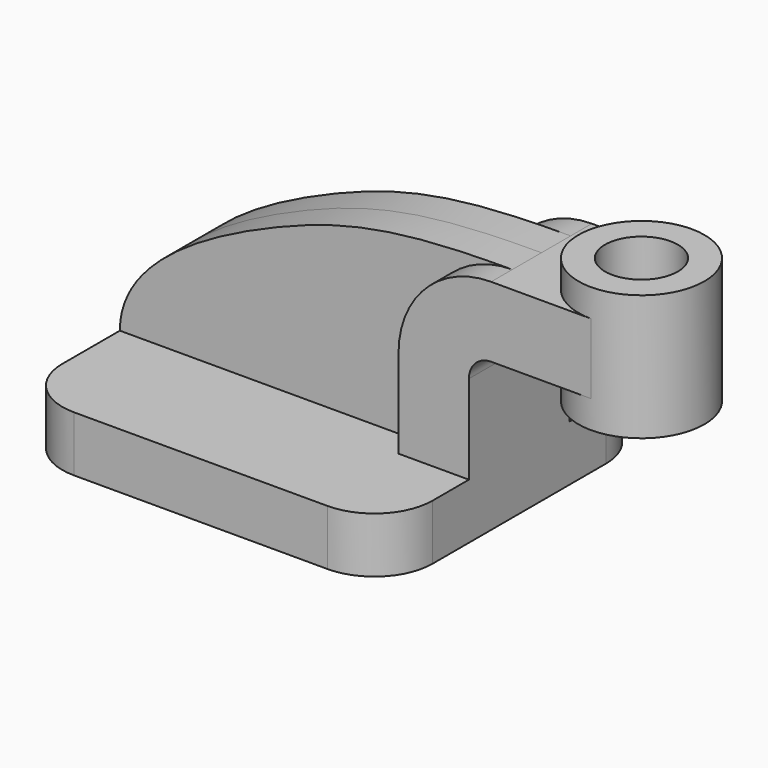
from build123d import *

# Parameters (mm, degrees)
F1_DEPTH     = 57.15
F0_W         = 21.59
F0_H         = 24.13
F2_DEPTH     = 21.59
F3_DEPTH     = 12.5
F5_R         = 12.5
F6_DEPTH     = 90.806
F7_R         = 20
F8_T         = 2.5
F8_T3_DEPTH  = 107.87
F8_T5_DEPTH  = 14.09
F8_T7_DEPTH  = 29.13
F8_T9_DEPTH  = 14.09
F8_T11_DEPTH = 35.48
F8_T14_ANGLE = 90.000000001
F8_T16_ANGLE = 90.000000001
F8_T18_ANGLE = 180.000000001
F8_T20_ANGLE = 180.000000001


# Not quite as in the source:
# - a shell that OpenCascade refuses in one call is made with other operations: the cavity is built on its own and cut out


with BuildPart() as f1:
    # F0 (on Front) → F1 (new body, symmetric)
    with BuildSketch(Plane.XZ):
        Polygon((-63.5, -9.525), (63.5, -9.525), (63.5, 9.525), (39.37, 9.525), (-63.5, 9.525), align=None)
    extrude(amount=F1_DEPTH, both=True)

    # F0 (on Front) → F2 (join, symmetric)
    with BuildSketch(Plane.XZ):
        with BuildLine():
            Line((39.37, 9.525), (63.5, 9.525))
            Line((63.5, 9.525), (63.5, 40.005))
            ThreePointArc((63.5, 40.005), (65.7318463274, 45.3931536726), (71.12, 47.625))
            Line((71.12, 47.625), (83.82, 47.625))
            Line((83.82, 47.625), (83.82, 71.755))
            Line((83.82, 71.755), (71.12, 71.755))
            ThreePointArc((71.12, 71.755), (48.6693596973, 62.4556403027), (39.37, 40.005))
            Line((39.37, 40.005), (39.37, 9.525))
        make_face()
        with Locations((94.615, 59.69)):
            Rectangle(F0_W, F0_H)
    extrude(amount=F2_DEPTH, both=True)

    # F0 (on Front) → F3 (join, symmetric)
    with BuildSketch(Plane.XZ):
        with BuildLine():
            add(Edge.make_bspline(
                [(-63.5, 9.525), (-63.5, 31.5907289062), (-3.4680848518, 65.1337229979), (32.8965573805, 71.755), (71.12, 71.755)],
                knots=[0, 0, 0, 0, 0.4791248693, 1, 1, 1, 1], degree=3))
            Line((-63.5, 9.525), (39.37, 9.525))
            Line((39.37, 9.525), (39.37, 40.005))
            ThreePointArc((39.37, 40.005), (48.6693596973, 62.4556403027), (71.12, 71.755))
        make_face()
    extrude(amount=F3_DEPTH, both=True)

    # F0 (on Front) → F4 (revolve)
    with BuildSketch(Plane.XZ):
        Polygon((105.41, 81.28), (105.41, 71.755), (105.41, 47.625), (105.41, 38.1), (127, 38.1), (127, 81.28), align=None)
    revolve(axis=Axis((105.41, 0, 59.69), (0, 0, -1)))

    # F5 (on face) → F6 (cut, through all)
    with BuildSketch(Plane.XY.offset(81.28)):
        with Locations((105.41, 0)):
            Circle(F5_R)
    extrude(amount=-F6_DEPTH, mode=Mode.SUBTRACT)

    # F7
    f7_edges = [f1.edges().sort_by_distance(p)[0] for p in [
        (63.5, -57.15, 0),
        (-63.5, -57.15, 0),
        (63.5, 57.15, 0),
        (-63.5, 57.15, 0),
    ]]
    fillet(f7_edges, radius=F7_R)

    # F8: shell of thickness 2.5, made by hand


with BuildPart() as f8_core1:
    # F8_t2: copy of F1
    add(f1.part)

    # the walls: a layer under each face that stays
    f8_faces = [f8_core1.faces().sort_by_distance(p)[0] for p in [
        (0, 57.15, 0),
        (-57.6421356237, 51.2921356237, 0),
        (57.6421356237, 51.2921356237, 0),
        (-63.5, 0, 0),
        (63.5, 0, 15.24),
        (-57.6421356237, -51.2921356237, 0),
        (57.6421356237, -51.2921356237, 0),
        (0, -57.15, 0),
        (0, 34.825, 9.525),
        (0, -34.825, 9.525),
        (-8.3874166975, -6.25, 58.8110273922),
        (-8.3874166975, 6.25, 58.8110273922),
        (50.3766666667, 21.59, 19.8966666667),
        (50.3766666667, -21.59, 19.8966666667),
        (65.7318463274, 0, 45.3931536726),
        (3.81, 12.5, 40.64),
        (39.37, 17.045, 24.765),
        (3.81, -12.5, 40.64),
        (39.37, -17.045, 24.765),
        (88.265, 14.3933333333, 71.755),
        (76.835, 14.3933333333, 47.625),
        (116.205, -18.6974884677, 45.2966666667),
        (48.6693596973, 17.045, 62.4556403027),
        (48.6693596973, -17.045, 62.4556403027),
        (91.0166666667, 14.3933333333, 81.28),
        (119.8033333333, 14.3933333333, 38.1),
        (92.91, 0, 59.69),
    ]]
    thicken(f8_faces, amount=-F8_T, mode=Mode.SUBTRACT)

    # F8_s4 → F8_t3 (cut)
    with BuildSketch(Plane.YZ.offset(-66)):
        Polygon((12.525, 9.55), (12.5, 7.025), (10, 7.025), (10, 9.525), align=None)
        Polygon((-12.525, 9.55), (-12.5, 7.025), (-10, 7.025), (-10, 9.525), align=None)
    extrude(amount=F8_T3_DEPTH, mode=Mode.SUBTRACT)

    # F8_s6 → F8_t5 (cut)
    with BuildSketch(Plane.XZ.offset(-24.09)):
        Polygon((39.345, 9.55), (39.37, 7.025), (41.87, 7.025), (41.87, 9.525), align=None)
    extrude(amount=F8_T5_DEPTH, mode=Mode.SUBTRACT)

    # F8_s8 → F8_t7 (cut)
    with BuildSketch(Plane.YZ.offset(36.87)):
        Polygon((21.615, 9.55), (21.59, 7.025), (19.09, 7.025), (19.09, 9.525), align=None)
        Polygon((-21.615, 9.55), (-21.59, 7.025), (-19.09, 7.025), (-19.09, 9.525), align=None)
    extrude(amount=F8_T7_DEPTH, mode=Mode.SUBTRACT)

    # F8_s10 → F8_t9 (cut)
    with BuildSketch(Plane.XZ.offset(10)):
        Polygon((39.345, 9.55), (39.37, 7.025), (41.87, 7.025), (41.87, 9.525), align=None)
    extrude(amount=F8_T9_DEPTH, mode=Mode.SUBTRACT)

    # F8_s12 → F8_t11 (cut)
    with BuildSketch(Plane.XY.offset(7.025)):
        Polygon((39.345, 12.525), (39.37, 10), (41.87, 10), (41.87, 12.5), align=None)
        Polygon((39.345, -12.525), (39.37, -10), (41.87, -10), (41.87, -12.5), align=None)
    extrude(amount=F8_T11_DEPTH, mode=Mode.SUBTRACT)

    # F8_s13 → F8_t14 (revolve, cut)
    with BuildSketch(Plane.XY.offset(40.005)):
        Polygon((39.345, 12.525), (39.37, 10), (41.87, 10), (41.87, 12.5), align=None)
    revolve(axis=Axis((71.12, 12.5, 40.005), (0, 1, 0)), revolution_arc=F8_T14_ANGLE, mode=Mode.SUBTRACT)

    # F8_s15 → F8_t16 (revolve, cut)
    with BuildSketch(Plane.XY.offset(40.005)):
        Polygon((39.345, -12.525), (39.37, -10), (41.87, -10), (41.87, -12.5), align=None)
    revolve(axis=Axis((71.12, -12.5, 40.005), (0, 1, 0)), revolution_arc=F8_T16_ANGLE, mode=Mode.SUBTRACT)

    # F8_s17 → F8_t18 (revolve, cut)
    with BuildSketch(Plane.YZ.offset(105.41)):
        Polygon((21.615, 71.78), (21.59, 69.255), (19.09, 69.255), (19.09, 71.755), align=None)
    revolve(axis=Axis((105.41, 0, 71.755), (0, 0, 1)), revolution_arc=F8_T18_ANGLE, mode=Mode.SUBTRACT)

    # F8_s19 → F8_t20 (revolve, cut)
    with BuildSketch(Plane.YZ.offset(105.41)):
        Polygon((21.615, 47.6), (21.59, 50.125), (19.09, 50.125), (19.09, 47.625), align=None)
    revolve(axis=Axis((105.41, 0, 47.625), (0, 0, 1)), revolution_arc=F8_T20_ANGLE, mode=Mode.SUBTRACT)


with BuildPart() as f1_1:
    add(f1.part)

    # what is left inside the walls is the cavity
    f8_cavity = [f8_core1.part.solids().sort_by_distance(p)[0] for p in [
        (0, 18.216667, -9.5),
    ]]
    add(f8_cavity, mode=Mode.SUBTRACT)


solid = f1_1.part
